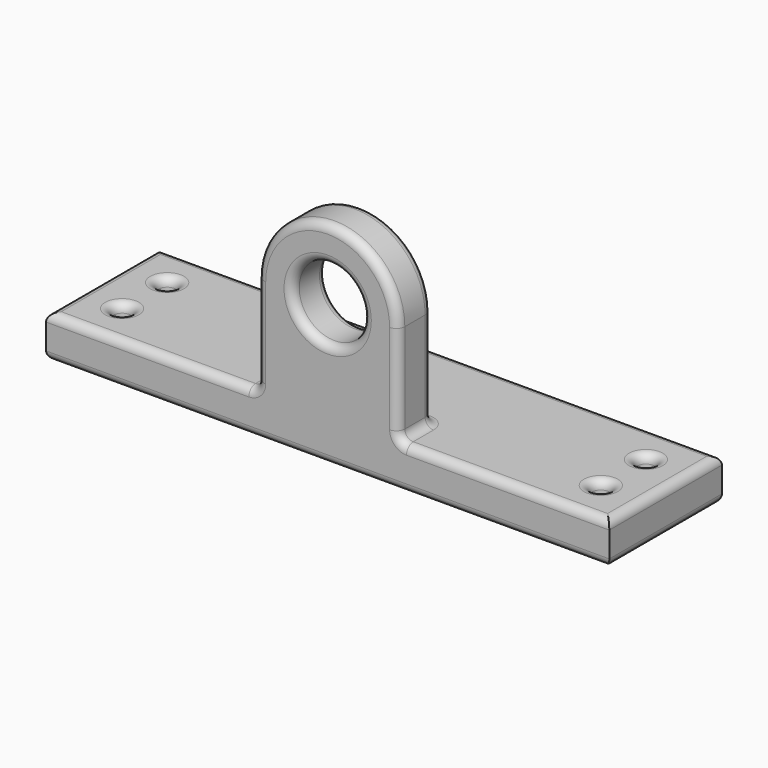
from build123d import *

# Parameters (mm, degrees)
F0_W     = 200
F0_H     = 50
F0_R     = 3
F1_DEPTH = 15
F2_W     = 50
F2_H     = 15
F3_DEPTH = 15
F4_R     = 3


with BuildPart() as f1:
    # F0 (on Top) → F1 (new body)
    with BuildSketch(Plane.XY):
        Rectangle(F0_W, F0_H)
        with Locations((-85, -10)):
            Circle(F0_R, mode=Mode.SUBTRACT)
        with Locations((85, -10)):
            Circle(F0_R, mode=Mode.SUBTRACT)
        with Locations((-85, 10)):
            Circle(F0_R, mode=Mode.SUBTRACT)
        with Locations((85, 10)):
            Circle(F0_R, mode=Mode.SUBTRACT)
    extrude(amount=F1_DEPTH)

    # F2 (on face) → F3 (join)
    with BuildSketch(Plane.XZ.offset(25)):
        with BuildLine():
            Line((12.5, 50), (25, 50))
            ThreePointArc((25, 50), (0, 75), (-25, 50))
            Line((-25, 50), (-12.5, 50))
            ThreePointArc((-12.5, 50), (0, 62.5), (12.5, 50))
        make_face()
        with BuildLine():
            ThreePointArc((-25, 50), (0, 25), (25, 50))
            Line((25, 50), (12.5, 50))
            ThreePointArc((12.5, 50), (0, 37.5), (-12.5, 50))
            Line((-12.5, 50), (-25, 50))
        make_face()
        with BuildLine():
            Line((25, 15), (25, 50))
            ThreePointArc((25, 50), (0, 25), (-25, 50))
            Line((-25, 50), (-25, 15))
            Line((-25, 15), (25, 15))
        make_face()
        with Locations((0, 7.5)):
            Rectangle(F2_W, F2_H)
    extrude(amount=-F3_DEPTH)

    # F4
    f4_edges = [f1.edges().sort_by_distance(p)[0] for p in [
        (62.5, -25, 15),
        (25, -17.5, 15),
        (0, -10, 15),
        (-25, -17.5, 15),
        (-62.5, -25, 15),
        (-100, 0, 15),
        (0, 25, 15),
        (100, 0, 15),
        (-88, -10, 15),
        (82, -10, 15),
        (-88, 10, 15),
        (82, 10, 15),
        (25, -10, 32.5),
        (-25, -10, 32.5),
        (0, -10, 75),
        (-12.5, -10, 50),
        (-12.5, -25, 50),
        (100, 0, 0),
        (0, 25, 0),
        (-100, 0, 0),
        (0, -25, 0),
        (-88, -10, 0),
        (82, -10, 0),
        (-88, 10, 0),
        (82, 10, 0),
        (-25, -25, 32.5),
        (0, -25, 75),
        (25, -25, 32.5),
    ]]
    fillet(f4_edges, radius=F4_R)


solid = f1.part
